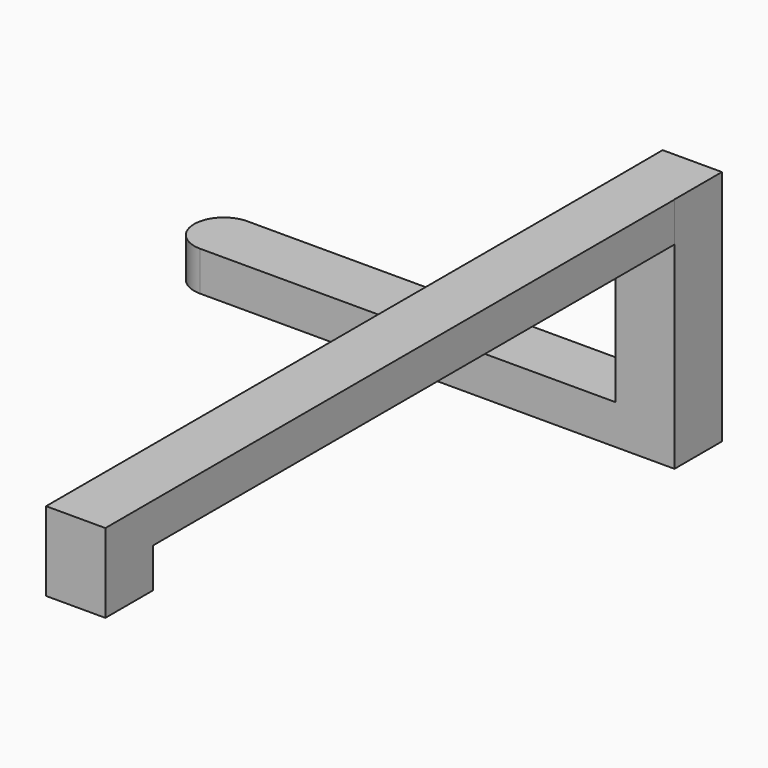
from build123d import *

# Parameters (mm, degrees)
F1_DEPTH = 12.7
F2_DEPTH = 76.2
F4_DEPTH = 12.7
F3_W     = 19.05
F3_H     = 19.05
F5_DEPTH = 25.4


# Not quite as in the source:
# - a feature names something its author has since deleted; it is built from what else it names


with BuildPart() as f1:
    # F0 (on Top) → F1 (new body)
    with BuildSketch(Plane.XY):
        with BuildLine():
            Line((59.8826112453, 4.7625), (-73.4673887547, 4.7625))
            ThreePointArc((-73.4673887547, 4.7625), (-82.9923886673, -4.7625000437), (-73.4673886673, -14.2875))
            Line((-73.4673886673, -14.2875), (59.9451471992, -14.2875))
            Line((59.9451471992, -14.2875), (59.8826112453, 4.7625))
        make_face()
        Polygon((78.9326112453, 4.7625), (59.8826112453, 4.7625), (59.9451471992, -14.2875), (78.9326113327, -14.2875), align=None)
    extrude(amount=F1_DEPTH)

    # F0 (on Top) → F2 (join)
    with BuildSketch(Plane.XY):
        Polygon((78.9326112453, 4.7625), (59.8826112453, 4.7625), (59.9451471992, -14.2875), (78.9326113327, -14.2875), align=None)
    extrude(amount=F2_DEPTH)

    # F3 (on face) → F4 (join)
    with BuildSketch(Plane.XY.offset(76.2)):
        Polygon((78.9326113327, -14.2875), (59.9451471992, -14.2875), (59.9451471992, -223.8375), (78.9951471992, -223.8375), (78.9951471992, -14.2875), align=None)
    extrude(amount=-F4_DEPTH)

    # F3 (on face) → F5 (join)
    with BuildSketch(Plane.XY.offset(76.2)):
        with Locations((69.4701471992, -233.3625)):
            Rectangle(F3_W, F3_H)
    extrude(amount=-F5_DEPTH)


with BuildPart() as f6_1:
    # F6: copy of F1
    add(f1.part)


solid = f1.part
